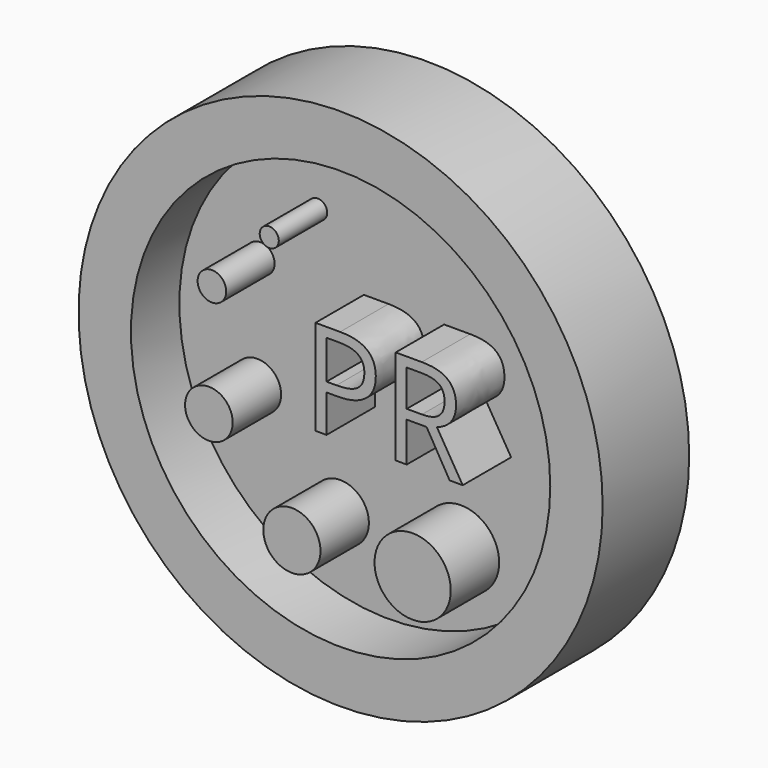
from build123d import *

# Parameters (mm, degrees)
F0_R         = 27.5
F0_R_2       = 22
F0_R_3       = 1
F0_R_4       = 1.5
F0_R_5       = 2.5
F0_R_6       = 3
F0_R_7       = 4
F0_TEXT_SIZE = 13.9830504648
F1_DEPTH     = 6.35
F2_R         = 27.5
F3_DEPTH     = 5


# Not quite as in the source:
# - Text() gives the source's letters only with a copy of the font that has no kerning and outlines rounded to 1/6400 em; it was checked with that copy


with BuildPart() as f1:
    # F0 (on Front) → F1 (new body)
    with BuildSketch(Plane.XZ):
        Circle(F0_R)
        Circle(F0_R_2, mode=Mode.SUBTRACT)
        with Locations((-7.4874670245, 13.4338801727)):
            Circle(F0_R_3)
        with Locations((-13.5061163455, 6.9400751963)):
            Circle(F0_R_4)
        with Locations((-13.8228880242, -4.9388385378)):
            Circle(F0_R_5)
        with Locations((-5.1116850227, -13.8084273785)):
            Circle(F0_R_6)
        with Locations((7.5591569766, -13.016499579)):
            Circle(F0_R_7)
        with Locations((-4.0102573112, -2.8813069221)):
            Text('PR', F0_TEXT_SIZE, font='Open Sans', text_align=(TextAlign.LEFT, TextAlign.BOTTOM))
    extrude(amount=F1_DEPTH)

    # F2 (on Front) → F3 (join)
    with BuildSketch(Plane.XZ):
        Circle(F2_R)
    extrude(amount=-F3_DEPTH)


solid = f1.part
